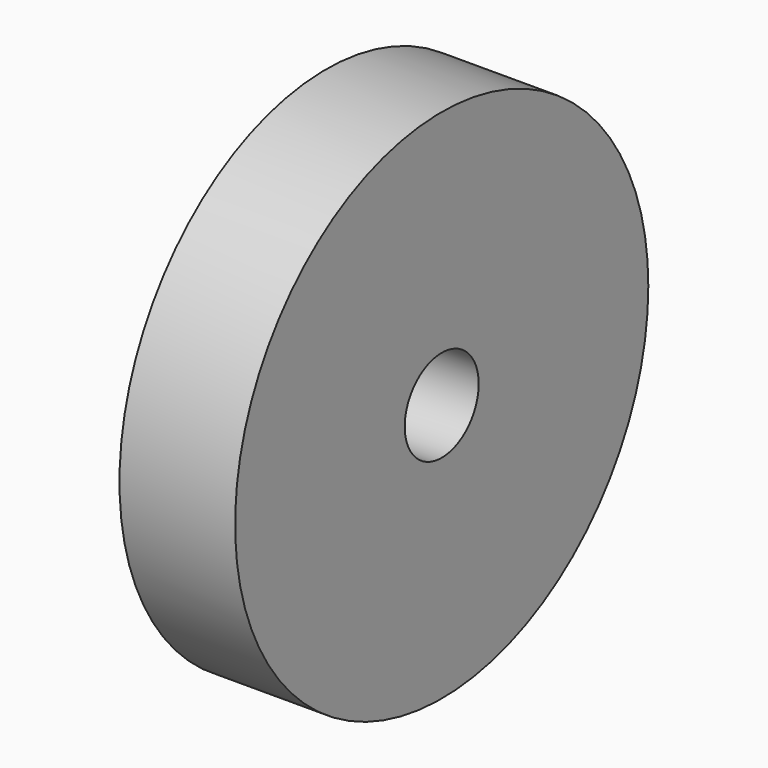
from build123d import *

# Parameters (mm, degrees)
F0_W = 1.5
F0_H = 2.75


with BuildPart() as f1:
    # F0 (on Top) → F1 (revolve)
    with BuildSketch(Plane.XY):
        with Locations((0.75, 1.975)):
            Rectangle(F0_W, F0_H)
    revolve(axis=Axis((0.75, 0, 0), (1, 0, 0)))


solid = f1.part
